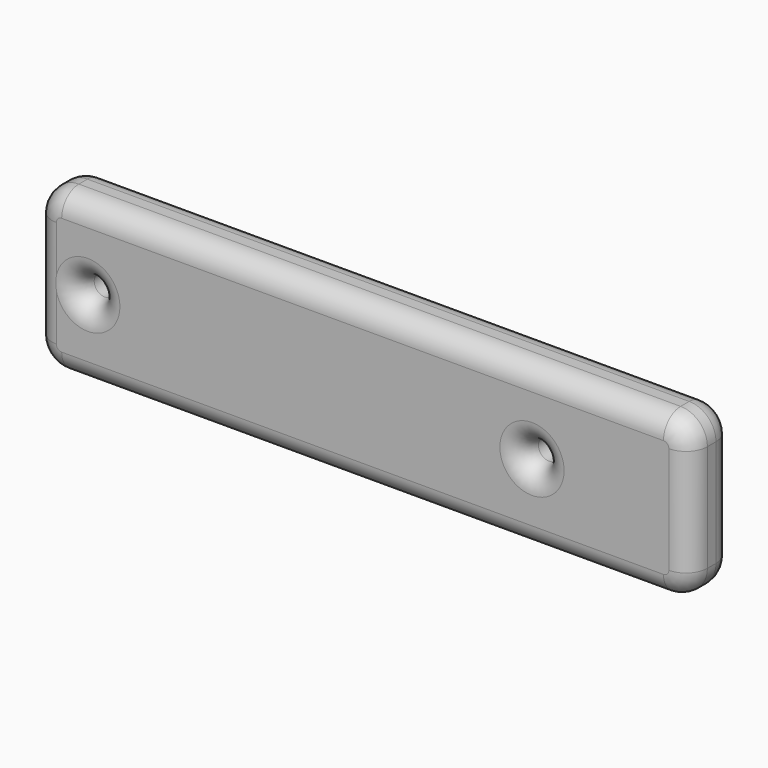
from build123d import *

# Parameters (mm, degrees)
F0_R         = 2.54
F1_DEPTH     = 12.7
F2_T1_DEPTH  = 142.748
F2_T3_DEPTH  = 25.4
F2_T6_ANGLE  = 90
F2_T8_ANGLE  = 90
F2_T10_ANGLE = 90
F2_T12_ANGLE = 90
F2_T18_ANGLE = 90
F2_T20_ANGLE = 90
F2_T22_ANGLE = 90
F2_T24_ANGLE = 90


# Not quite as in the source:
# - a fillet or chamfer that OpenCascade refuses, or shapes differently, is made with other operations: its cross-section is extruded or revolved along the edge and cut away or added


with BuildPart() as f1:
    # F0 (on Front) → F1 (new body)
    with BuildSketch(Plane.XZ):
        with BuildLine():
            Line((70.9908799698, 13.4507374847), (-71.7571200302, 13.4507374847))
            ThreePointArc((-71.7571200302, 13.4507374847), (-76.2472480907, 11.5908655453), (-78.1071200302, 7.1007374847))
            Line((-78.1071200302, 7.1007374847), (-78.1071200302, -18.2992625153))
            ThreePointArc((-78.1071200302, -18.2992625153), (-76.2472480907, -22.7893905758), (-71.7571200302, -24.6492625153))
            Line((-71.7571200302, -24.6492625153), (70.9908799698, -24.6492625153))
            ThreePointArc((70.9908799698, -24.6492625153), (75.4810080304, -22.7893905758), (77.3408799698, -18.2992625153))
            Line((77.3408799698, -18.2992625153), (77.3408799698, 7.1007374847))
            ThreePointArc((77.3408799698, 7.1007374847), (75.4810080304, 11.5908655453), (70.9908799698, 13.4507374847))
        make_face()
        with Locations((-65.5671200302, -5.5992625153)):
            Circle(F0_R, mode=Mode.SUBTRACT)
        with Locations((39.8008799698, -5.5992626585)):
            Circle(F0_R, mode=Mode.SUBTRACT)
    extrude(amount=F1_DEPTH)

    # F2: fillet of radius 5.08 on 20 edges, made by hand

    # F2_s2 → F2_t1 (cut)
    with BuildSketch(Plane.YZ.offset(-71.7571200302)):
        with BuildLine():
            ThreePointArc((-7.62, 13.4507374847), (-11.2121024484, 11.9628399332), (-12.7, 8.3707374847))
            Line((-12.7, 8.3707374847), (-12.7, 13.4507374847))
            Line((-12.7, 13.4507374847), (-7.62, 13.4507374847))
        make_face()
        with BuildLine():
            ThreePointArc((-5.08, 13.4507374847), (-1.4878975516, 11.9628399332), (0, 8.3707374847))
            Line((0, 8.3707374847), (0, 13.4507374847))
            Line((0, 13.4507374847), (-5.08, 13.4507374847))
        make_face()
        with BuildLine():
            ThreePointArc((-7.62, -24.6492625153), (-11.2121024484, -23.1613649637), (-12.7, -19.5692625153))
            Line((-12.7, -19.5692625153), (-12.7, -24.6492625153))
            Line((-12.7, -24.6492625153), (-7.62, -24.6492625153))
        make_face()
        with BuildLine():
            ThreePointArc((-5.08, -24.6492625153), (-1.4878975516, -23.1613649637), (0, -19.5692625153))
            Line((0, -19.5692625153), (0, -24.6492625153))
            Line((0, -24.6492625153), (-5.08, -24.6492625153))
        make_face()
    extrude(amount=F2_T1_DEPTH, mode=Mode.SUBTRACT)

    # F2_s4 → F2_t3 (cut)
    with BuildSketch(Plane.XY.offset(-18.2992625153)):
        with BuildLine():
            ThreePointArc((-78.1071200302, -5.08), (-76.6192224786, -1.4878975516), (-73.0271200302, 0))
            Line((-73.0271200302, 0), (-78.1071200302, 0))
            Line((-78.1071200302, 0), (-78.1071200302, -5.08))
        make_face()
        with BuildLine():
            ThreePointArc((77.3408799698, -5.08), (75.8529824183, -1.4878975516), (72.2608799698, 0))
            Line((72.2608799698, 0), (77.3408799698, 0))
            Line((77.3408799698, 0), (77.3408799698, -5.08))
        make_face()
        with BuildLine():
            ThreePointArc((-78.1071200302, -7.62), (-76.6192224786, -11.2121024484), (-73.0271200302, -12.7))
            Line((-73.0271200302, -12.7), (-78.1071200302, -12.7))
            Line((-78.1071200302, -12.7), (-78.1071200302, -7.62))
        make_face()
        with BuildLine():
            ThreePointArc((77.3408799698, -7.62), (75.8529824183, -11.2121024484), (72.2608799698, -12.7))
            Line((72.2608799698, -12.7), (77.3408799698, -12.7))
            Line((77.3408799698, -12.7), (77.3408799698, -7.62))
        make_face()
    extrude(amount=F2_T3_DEPTH, mode=Mode.SUBTRACT)

    # F2_s5 → F2_t6 (revolve, cut)
    with BuildSketch(Plane.YZ.offset(-71.7571200302)):
        with BuildLine():
            ThreePointArc((-5.08, 13.4507374847), (-1.4878975516, 11.9628399332), (0, 8.3707374847))
            Line((0, 8.3707374847), (0, 13.4507374847))
            Line((0, 13.4507374847), (-5.08, 13.4507374847))
        make_face()
    revolve(axis=Axis((-71.7571200302, 0, 7.1007374847), (0, -1, 0)), revolution_arc=F2_T6_ANGLE, mode=Mode.SUBTRACT)

    # F2_s7 → F2_t8 (revolve, cut)
    with BuildSketch(Plane.XY.offset(-18.2992625153)):
        with BuildLine():
            ThreePointArc((-78.1071200302, -5.08), (-76.6192224786, -1.4878975516), (-73.0271200302, 0))
            Line((-73.0271200302, 0), (-78.1071200302, 0))
            Line((-78.1071200302, 0), (-78.1071200302, -5.08))
        make_face()
    revolve(axis=Axis((-71.7571200302, 0, -18.2992625153), (0, -1, 0)), revolution_arc=F2_T8_ANGLE, mode=Mode.SUBTRACT)

    # F2_s9 → F2_t10 (revolve, cut)
    with BuildSketch(Plane.YZ.offset(70.9908799698)):
        with BuildLine():
            ThreePointArc((-5.08, -24.6492625153), (-1.4878975516, -23.1613649637), (0, -19.5692625153))
            Line((0, -19.5692625153), (0, -24.6492625153))
            Line((0, -24.6492625153), (-5.08, -24.6492625153))
        make_face()
    revolve(axis=Axis((70.9908799698, 0, -18.2992625153), (0, -1, 0)), revolution_arc=F2_T10_ANGLE, mode=Mode.SUBTRACT)

    # F2_s11 → F2_t12 (revolve, cut)
    with BuildSketch(Plane.XY.offset(7.1007374847)):
        with BuildLine():
            ThreePointArc((77.3408799698, -5.08), (75.8529824183, -1.4878975516), (72.2608799698, 0))
            Line((72.2608799698, 0), (77.3408799698, 0))
            Line((77.3408799698, 0), (77.3408799698, -5.08))
        make_face()
    revolve(axis=Axis((70.9908799698, 0, 7.1007374847), (0, -1, 0)), revolution_arc=F2_T12_ANGLE, mode=Mode.SUBTRACT)

    # F2_s13 → F2_t14 (revolve, cut)
    with BuildSketch(Plane.XY.offset(-5.5992625153)):
        with BuildLine():
            ThreePointArc((-63.0271200302, -5.08), (-61.5392224786, -1.4878975516), (-57.9471200302, 0))
            Line((-57.9471200302, 0), (-63.0271200302, 0))
            Line((-63.0271200302, 0), (-63.0271200302, -5.08))
        make_face()
    revolve(axis=Axis((-65.5671200302, 0, -5.5992625153), (0, -1, 0)), mode=Mode.SUBTRACT)

    # F2_s15 → F2_t16 (revolve, cut)
    with BuildSketch(Plane.XY.offset(-5.5992626585)):
        with BuildLine():
            ThreePointArc((42.3408799698, -5.08), (43.8287775214, -1.4878975516), (47.4208799698, 0))
            Line((47.4208799698, 0), (42.3408799698, 0))
            Line((42.3408799698, 0), (42.3408799698, -5.08))
        make_face()
    revolve(axis=Axis((39.8008799698, 0, -5.5992626585), (0, -1, 0)), mode=Mode.SUBTRACT)

    # F2_s17 → F2_t18 (revolve, cut)
    with BuildSketch(Plane.YZ.offset(-71.7571200302)):
        with BuildLine():
            ThreePointArc((-7.62, 13.4507374847), (-11.2121024484, 11.9628399332), (-12.7, 8.3707374847))
            Line((-12.7, 8.3707374847), (-12.7, 13.4507374847))
            Line((-12.7, 13.4507374847), (-7.62, 13.4507374847))
        make_face()
    revolve(axis=Axis((-71.7571200302, -12.7, 7.1007374847), (0, -1, 0)), revolution_arc=F2_T18_ANGLE, mode=Mode.SUBTRACT)

    # F2_s19 → F2_t20 (revolve, cut)
    with BuildSketch(Plane.XY.offset(-18.2992625153)):
        with BuildLine():
            ThreePointArc((-78.1071200302, -7.62), (-76.6192224786, -11.2121024484), (-73.0271200302, -12.7))
            Line((-73.0271200302, -12.7), (-78.1071200302, -12.7))
            Line((-78.1071200302, -12.7), (-78.1071200302, -7.62))
        make_face()
    revolve(axis=Axis((-71.7571200302, -12.7, -18.2992625153), (0, -1, 0)), revolution_arc=F2_T20_ANGLE, mode=Mode.SUBTRACT)

    # F2_s21 → F2_t22 (revolve, cut)
    with BuildSketch(Plane.YZ.offset(70.9908799698)):
        with BuildLine():
            ThreePointArc((-7.62, -24.6492625153), (-11.2121024484, -23.1613649637), (-12.7, -19.5692625153))
            Line((-12.7, -19.5692625153), (-12.7, -24.6492625153))
            Line((-12.7, -24.6492625153), (-7.62, -24.6492625153))
        make_face()
    revolve(axis=Axis((70.9908799698, -12.7, -18.2992625153), (0, -1, 0)), revolution_arc=F2_T22_ANGLE, mode=Mode.SUBTRACT)

    # F2_s23 → F2_t24 (revolve, cut)
    with BuildSketch(Plane.XY.offset(7.1007374847)):
        with BuildLine():
            ThreePointArc((77.3408799698, -7.62), (75.8529824183, -11.2121024484), (72.2608799698, -12.7))
            Line((72.2608799698, -12.7), (77.3408799698, -12.7))
            Line((77.3408799698, -12.7), (77.3408799698, -7.62))
        make_face()
    revolve(axis=Axis((70.9908799698, -12.7, 7.1007374847), (0, -1, 0)), revolution_arc=F2_T24_ANGLE, mode=Mode.SUBTRACT)

    # F2_s25 → F2_t26 (revolve, cut)
    with BuildSketch(Plane.XY.offset(-5.5992625153)):
        with BuildLine():
            ThreePointArc((-63.0271200302, -7.62), (-61.5392224786, -11.2121024484), (-57.9471200302, -12.7))
            Line((-57.9471200302, -12.7), (-63.0271200302, -12.7))
            Line((-63.0271200302, -12.7), (-63.0271200302, -7.62))
        make_face()
    revolve(axis=Axis((-65.5671200302, -12.7, -5.5992625153), (0, -1, 0)), mode=Mode.SUBTRACT)

    # F2_s27 → F2_t28 (revolve, cut)
    with BuildSketch(Plane.XY.offset(-5.5992626585)):
        with BuildLine():
            ThreePointArc((42.3408799698, -7.62), (43.8287775214, -11.2121024484), (47.4208799698, -12.7))
            Line((47.4208799698, -12.7), (42.3408799698, -12.7))
            Line((42.3408799698, -12.7), (42.3408799698, -7.62))
        make_face()
    revolve(axis=Axis((39.8008799698, -12.7, -5.5992626585), (0, -1, 0)), mode=Mode.SUBTRACT)


solid = f1.part
